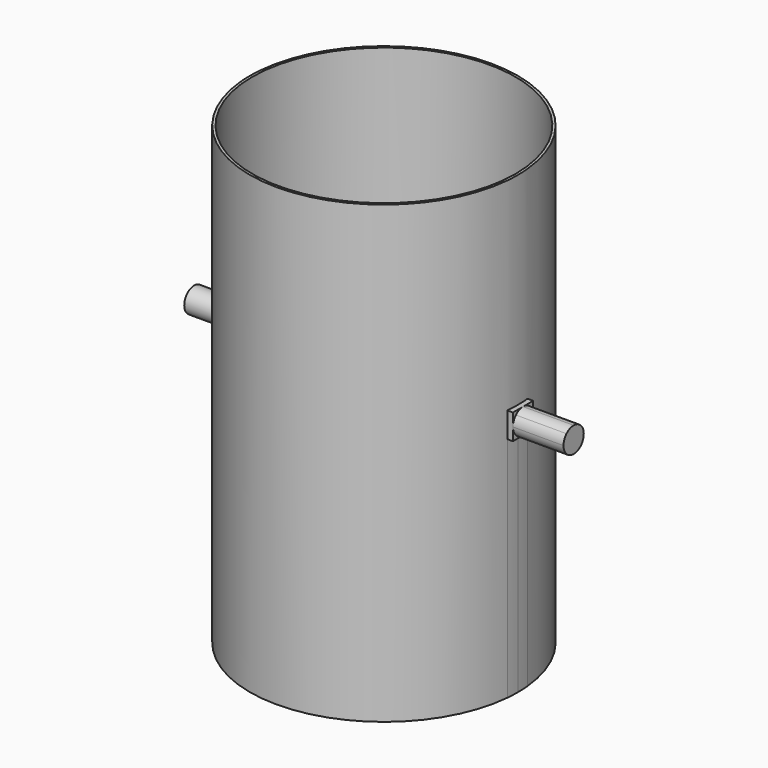
from build123d import *
from build123d import SkipClean  # not in build123d's __all__

# Parameters (mm, degrees)
F0_R     = 260
F1_DEPTH = 10
F2_DEPTH = 900
F3_DEPTH = 500
F4_DEPTH = 450
F5_R     = 24.5282559267
F6_DEPTH = 100
F8_DEPTH = 100


# Not quite as in the source:
# - after a boolean that leaves OpenCascade's solid faulty, fix() repairs it


with BuildPart() as f1:
    # F0 (on Top) → F1 (new body)
    with BuildSketch(Plane.XY):
        with BuildLine():
            ThreePointArc((263.8181191655, -25), (264.7043648855, -12.5139606271), (265, 0))
            ThreePointArc((265, 0), (264.7043648855, 12.5139606271), (263.8181191655, 25))
            ThreePointArc((263.8181191655, 25), (0, 265), (-263.8181191655, 25))
            ThreePointArc((-263.8181191655, 25), (-264.7043648855, 12.5139606271), (-265, 0))
            ThreePointArc((-265, 0), (-264.7043648855, -12.5139606271), (-263.8181191655, -25))
            ThreePointArc((-263.8181191655, -25), (0, -265), (263.8181191655, -25))
        make_face()
        Circle(F0_R, mode=Mode.SUBTRACT)
        Circle(F0_R)
    extrude(amount=F1_DEPTH)

    # F0 (on Top) → F2 (join)
    with BuildSketch(Plane.XY):
        with BuildLine():
            ThreePointArc((263.8181191655, -25), (264.7043648855, -12.5139606271), (265, 0))
            ThreePointArc((265, 0), (264.7043648855, 12.5139606271), (263.8181191655, 25))
            ThreePointArc((263.8181191655, 25), (0, 265), (-263.8181191655, 25))
            ThreePointArc((-263.8181191655, 25), (-264.7043648855, 12.5139606271), (-265, 0))
            ThreePointArc((-265, 0), (-264.7043648855, -12.5139606271), (-263.8181191655, -25))
            ThreePointArc((-263.8181191655, -25), (0, -265), (263.8181191655, -25))
        make_face()
        Circle(F0_R, mode=Mode.SUBTRACT)
    extrude(amount=F2_DEPTH)

    # F0 (on Top) → F3 (join)
    with BuildSketch(Plane.XY):
        with BuildLine():
            Line((275, 0), (265, 0))
            ThreePointArc((265, 0), (264.7043648855, -12.5139606271), (263.8181191655, -25))
            Line((263.8181191655, -25), (275, -25))
            Line((275, -25), (275, 0))
        make_face()
        with BuildLine():
            ThreePointArc((263.8181191655, 25), (264.7043648855, 12.5139606271), (265, 0))
            Line((265, 0), (275, 0))
            Line((275, 0), (275, 25))
            Line((275, 25), (263.8181191655, 25))
        make_face()
        with BuildLine():
            ThreePointArc((-265, 0), (-264.7043648855, 12.5139606271), (-263.8181191655, 25))
            Line((-263.8181191655, 25), (-275, 25))
            Line((-275, 25), (-275, 0))
            Line((-275, 0), (-265, 0))
        make_face()
        with BuildLine():
            Line((-275, -25), (-263.8181191655, -25))
            ThreePointArc((-263.8181191655, -25), (-264.7043648855, -12.5139606271), (-265, 0))
            Line((-265, 0), (-275, 0))
            Line((-275, 0), (-275, -25))
        make_face()
    extrude(amount=F3_DEPTH)

    # F0 (on Top) → F4 (cut)
    with BuildSketch(Plane.XY):
        with BuildLine():
            ThreePointArc((263.8181191655, 25), (264.7043648855, 12.5139606271), (265, 0))
            Line((265, 0), (275, 0))
            Line((275, 0), (275, 25))
            Line((275, 25), (263.8181191655, 25))
        make_face()
        with BuildLine():
            Line((275, 0), (265, 0))
            ThreePointArc((265, 0), (264.7043648855, -12.5139606271), (263.8181191655, -25))
            Line((263.8181191655, -25), (275, -25))
            Line((275, -25), (275, 0))
        make_face()
        with BuildLine():
            ThreePointArc((-265, 0), (-264.7043648855, 12.5139606271), (-263.8181191655, 25))
            Line((-263.8181191655, 25), (-275, 25))
            Line((-275, 25), (-275, 0))
            Line((-275, 0), (-265, 0))
        make_face()
        with BuildLine():
            Line((-275, -25), (-263.8181191655, -25))
            ThreePointArc((-263.8181191655, -25), (-264.7043648855, -12.5139606271), (-265, 0))
            Line((-265, 0), (-275, 0))
            Line((-275, 0), (-275, -25))
        make_face()
    with SkipClean():  # cleaning this boolean's faces spoils the solid; the shape is the same uncleaned
        extrude(amount=F4_DEPTH, mode=Mode.SUBTRACT)

    # F5 (on face) → F6 (join)
    with BuildSketch(Plane(origin=(-275, 0, 0), x_dir=(0, -1, 0), z_dir=(-1, 0, 0))):
        with Locations((0, 475)):
            Circle(F5_R)
    extrude(amount=F6_DEPTH)

    add(f1.part.fix(), mode=Mode.REPLACE)

    # F7 (on face) → F8 (join)
    with BuildSketch(Plane.YZ.offset(275)):
        with BuildLine():
            Line((17.6776695297, 492.6776695297), (0, 475))
            Line((0, 475), (17.6776695297, 457.3223304703))
            ThreePointArc((17.6776695297, 457.3223304703), (23.0969883128, 465.4329141909), (25, 475))
            ThreePointArc((25, 475), (23.0969883128, 484.5670858091), (17.6776695297, 492.6776695297))
        make_face()
        with BuildLine():
            ThreePointArc((2.731e-07, 500), (-9.567085683, 498.096988365), (-17.6776695297, 492.6776695297))
            Line((-17.6776695297, 492.6776695297), (0, 475))
            Line((0, 475), (17.6776695297, 492.6776695297))
            ThreePointArc((17.6776695297, 492.6776695297), (9.5670859353, 498.0969882605), (2.731e-07, 500))
        make_face()
        with BuildLine():
            Line((0, 475), (-17.6776695297, 492.6776695297))
            ThreePointArc((-17.6776695297, 492.6776695297), (-23.0969883128, 484.5670858091), (-25, 475))
            ThreePointArc((-25, 475), (-23.0969883128, 465.4329141909), (-17.6776695297, 457.3223304703))
            Line((-17.6776695297, 457.3223304703), (0, 475))
        make_face()
        with BuildLine():
            Line((17.6776695297, 457.3223304703), (0, 475))
            Line((0, 475), (-17.6776695297, 457.3223304703))
            ThreePointArc((-17.6776695297, 457.3223304703), (-9.5670857461, 451.9030116611), (1.365e-07, 450))
            ThreePointArc((1.365e-07, 450), (9.5670858722, 451.9030117133), (17.6776695297, 457.3223304703))
        make_face()
    extrude(amount=F8_DEPTH)


solid = f1.part
